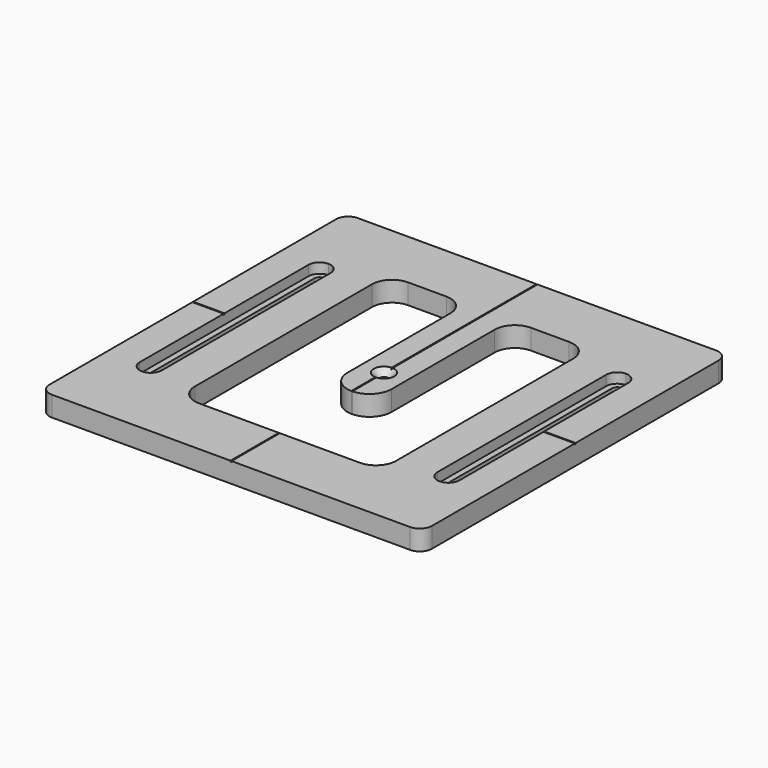
from build123d import *

# Parameters (mm, degrees)
F0_W         = 190
F0_H         = 190
F0_W_2       = 11
F0_H_2       = 115.8
F0_R         = 2.1
F0_W_3       = 0.5
F0_H_3       = 0.5
F1_DEPTH     = 10
F0_W_4       = 5.2
F0_H_4       = 110
F2_DEPTH     = 5
F3_R         = 2.59999
F4_R         = 5.49999
F6_DEPTH     = 25
F8_R         = 6
F7_W         = 0.5
F7_H         = 29.5
F9_DEPTH     = 0.5
F7_W_2       = 15.563522011
F7_H_2       = 0.5
F10_DEPTH    = 0.5
F11_T2_ANGLE = 359.64
F11_T4_ANGLE = 293.7301704478
F11_T6_ANGLE = 293.7301704478


# Not quite as in the source:
# - a fillet or chamfer that OpenCascade refuses, or shapes differently, is made with other operations: its cross-section is extruded or revolved along the edge and cut away or added
# - a fillet or chamfer is up to 0.001 mm smaller than in the source, because OpenCascade refuses the exact size
# - ends of sketch curves that miss each other by under 0.0002 mm in the source are joined


with BuildPart() as f1:
    # F0 (on Top) → F1 (new body)
    with BuildSketch(Plane.XY):
        Rectangle(F0_W, F0_H)
        with BuildLine():
            ThreePointArc((50, -55), (47.0710678119, -62.0710678119), (40, -65))
            Line((40, -65), (0.25, -65))
            Line((0.25, -65), (0.25, -65.5))
            Line((0.25, -65.5), (-0.25, -65.5))
            Line((-0.25, -65.5), (-0.25, -65))
            Line((-0.25, -65), (-40, -65))
            ThreePointArc((-40, -65), (-47.0710678119, -62.0710678119), (-50, -55))
            Line((-50, -55), (-50, 55))
            ThreePointArc((-50, 55), (-47.0710678119, 62.0710678119), (-40, 65))
            Line((-40, 65), (-21, 65))
            ThreePointArc((-21, 65), (-13.9289321881, 62.0710678119), (-11, 55))
            Line((-11, 55), (-11, -9))
            ThreePointArc((-11, -9), (-7.8660663613, -16.6892782496), (-0.25, -19.997158724))
            Line((-0.25, -19.997158724), (-0.25, -19.5))
            Line((-0.25, -19.5), (0.25, -19.5))
            Line((0.25, -19.5), (0.25, -19.997158724))
            ThreePointArc((0.25, -19.997158724), (7.8660663613, -16.6892782496), (11, -9))
            Line((11, -9), (11, 55))
            ThreePointArc((11, 55), (13.9289321881, 62.0710678119), (21, 65))
            Line((21, 65), (40, 65))
            ThreePointArc((40, 65), (47.0710678119, 62.0710678119), (50, 55))
            Line((50, 55), (50, -55))
        make_face(mode=Mode.SUBTRACT)
        with Locations((-73.936477989, 0)):
            Rectangle(F0_W_2, F0_H_2, mode=Mode.SUBTRACT)
        Circle(F0_R, mode=Mode.SUBTRACT)
        with Locations((73.936477989, 0)):
            Rectangle(F0_W_2, F0_H_2, mode=Mode.SUBTRACT)
        with BuildLine():
            ThreePointArc((0, -20), (0.1250080726, -19.9992896581), (0.25, -19.997158724))
            Line((0.25, -19.997158724), (0.25, -19.5))
            Line((0.25, -19.5), (-0.25, -19.5))
            Line((-0.25, -19.5), (-0.25, -19.997158724))
            ThreePointArc((-0.25, -19.997158724), (-0.1250080726, -19.9992896581), (0, -20))
        make_face()
        with Locations((0, -65.25)):
            Rectangle(F0_W_3, F0_H_3)
    extrude(amount=F1_DEPTH)

    # F0 (on Top) → F2 (join)
    with BuildSketch(Plane.XY):
        with Locations((-73.936477989, 0)):
            Rectangle(F0_W_2, F0_H_2)
        with Locations((-73.936477989, 0)):
            Rectangle(F0_W_4, F0_H_4, mode=Mode.SUBTRACT)
        with Locations((73.936477989, 0)):
            Rectangle(F0_W_2, F0_H_2)
        with Locations((73.936477989, 0)):
            Rectangle(F0_W_4, F0_H_4, mode=Mode.SUBTRACT)
    extrude(amount=F2_DEPTH)

    # F3 (radius 2.6 in the source; OpenCascade refuses exactly that, so slightly less here)
    f3_edges = [f1.edges().sort_by_distance(p)[0] for p in [
        (-76.536478, 55, 2.5),
        (-71.336478, 55, 2.5),
        (-76.536478, -55, 2.5),
        (-71.336478, -55, 2.5),
        (76.536478, -55, 2.5),
        (71.336478, -55, 2.5),
        (71.336478, 55, 2.5),
        (76.536478, 55, 2.5),
    ]]
    fillet(f3_edges, radius=F3_R)

    # F4 (radius 5.5 in the source; OpenCascade refuses exactly that, so slightly less here)
    f4_edges = [f1.edges().sort_by_distance(p)[0] for p in [
        (-79.436478, 57.9, 7.5),
        (-68.436478, 57.9, 7.5),
        (79.436478, 57.9, 7.5),
        (68.436478, 57.9, 7.5),
        (68.436478, -57.9, 7.5),
        (79.436478, -57.9, 7.5),
        (-79.436478, -57.9, 7.5),
        (-68.436478, -57.9, 7.5),
    ]]
    fillet(f4_edges, radius=F4_R)

    # F5 (on face) → F6 (cut)
    with BuildSketch(Plane.XY.offset(5)):
        with BuildLine():
            Line((-73.686477989, -55.5), (-73.686477989, -54.9879537784))
            ThreePointArc((-73.686477989, -54.9879537784), (-73.8113279558, -54.9969866984), (-73.936467989, -55))
            ThreePointArc((-73.936467989, -55), (-74.0616280221, -54.9969866984), (-74.186477989, -54.9879537784))
            Line((-74.186477989, -54.9879537784), (-74.186477989, -55.5))
            Line((-74.186477989, -55.5), (-73.686477989, -55.5))
        make_face()
        with BuildLine():
            ThreePointArc((-73.936467989, 55), (-73.8113279558, 54.9969866984), (-73.686477989, 54.9879537784))
            Line((-73.686477989, 54.9879537784), (-73.686477989, 55.5))
            Line((-73.686477989, 55.5), (-74.186477989, 55.5))
            Line((-74.186477989, 55.5), (-74.186477989, 54.9879537784))
            ThreePointArc((-74.186477989, 54.9879537784), (-74.0616280221, 54.9969866984), (-73.936467989, 55))
        make_face()
    extrude(amount=-F6_DEPTH, mode=Mode.SUBTRACT)

    # F8
    f8_edges = [f1.edges().sort_by_distance(p)[0] for p in [
        (-95, -95, 5),
        (95, -95, 5),
        (95, 95, 5),
        (-95, 95, 5),
    ]]
    fillet(f8_edges, radius=F8_R)

    # F7 (on face) → F9 (cut)
    with BuildSketch(Plane.XY.offset(10)):
        with BuildLine():
            Line((-0.25, 95), (-0.25, 2.0850659462))
            ThreePointArc((-0.25, 2.0850659462), (0, 2.1), (0.25, 2.0850659462))
            Line((0.25, 2.0850659462), (0.25, 95))
            Line((0.25, 95), (-0.25, 95))
        make_face()
        with BuildLine():
            Line((-0.25, -2.0850659462), (-0.25, -19.6))
            Line((-0.25, -19.6), (0.25, -19.6))
            Line((0.25, -19.6), (0.25, -2.0850659462))
            ThreePointArc((0.25, -2.0850659462), (0, -2.1), (-0.25, -2.0850659462))
        make_face()
        with Locations((0, -80.25)):
            Rectangle(F7_W, F7_H)
        with BuildLine():
            Line((-0.25, -0.25), (-0.25, -2.0850659462))
            ThreePointArc((-0.25, -2.0850659462), (0, -2.1), (0.25, -2.0850659462))
            Line((0.25, -2.0850659462), (0.25, -0.25))
            Line((0.25, -0.25), (-0.25, -0.25))
        make_face()
        with BuildLine():
            Line((-0.25, 2.0850659462), (-0.25, 0.25))
            Line((-0.25, 0.25), (0.25, 0.25))
            Line((0.25, 0.25), (0.25, 2.0850659462))
            ThreePointArc((0.25, 2.0850659462), (0, 2.1), (-0.25, 2.0850659462))
        make_face()
    extrude(amount=-F9_DEPTH, mode=Mode.SUBTRACT)

    # F7 (on face) → F10 (cut)
    with BuildSketch(Plane.XY.offset(10)):
        with Locations((87.2182389945, 0)):
            Rectangle(F7_W_2, F7_H_2)
        with Locations((-87.2182389945, 0)):
            Rectangle(F7_W_2, F7_H_2)
    extrude(amount=-F10_DEPTH, mode=Mode.SUBTRACT)

    # F11: chamfer of 3 on 3 edges, made by hand

    # F11_s1 → F11_t2 (revolve, cut)
    with BuildSketch(Plane(origin=(0, 0, 0), x_dir=(0, 0, 1), z_dir=(0.0031415875, -0.9999950652, 0))):
        Polygon((10, -5.1), (7, -2.1), (10, -2.1), align=None)
    revolve(axis=Axis((0, 0, 10), (0, 0, 1)), revolution_arc=F11_T2_ANGLE, mode=Mode.SUBTRACT)

    # F11_s3 → F11_t4 (revolve, cut)
    with BuildSketch(Plane(origin=(0, 0, 0), x_dir=(0, 0, 1), z_dir=(0.9154508113, -0.4024298847, 0))):
        Polygon((10, -5.1), (7, -2.1), (10, -2.1), align=None)
    revolve(axis=Axis((0, 0, 10), (0, 0, 1)), revolution_arc=F11_T4_ANGLE, mode=Mode.SUBTRACT)

    # F11_s5 → F11_t6 (revolve, cut)
    with BuildSketch(Plane.XZ):
        Polygon((5.1, 10), (2.1, 7), (2.1, 10), align=None)
    revolve(axis=Axis((0, 0, 10), (0, 0, 1)), revolution_arc=F11_T6_ANGLE, mode=Mode.SUBTRACT)


solid = f1.part
